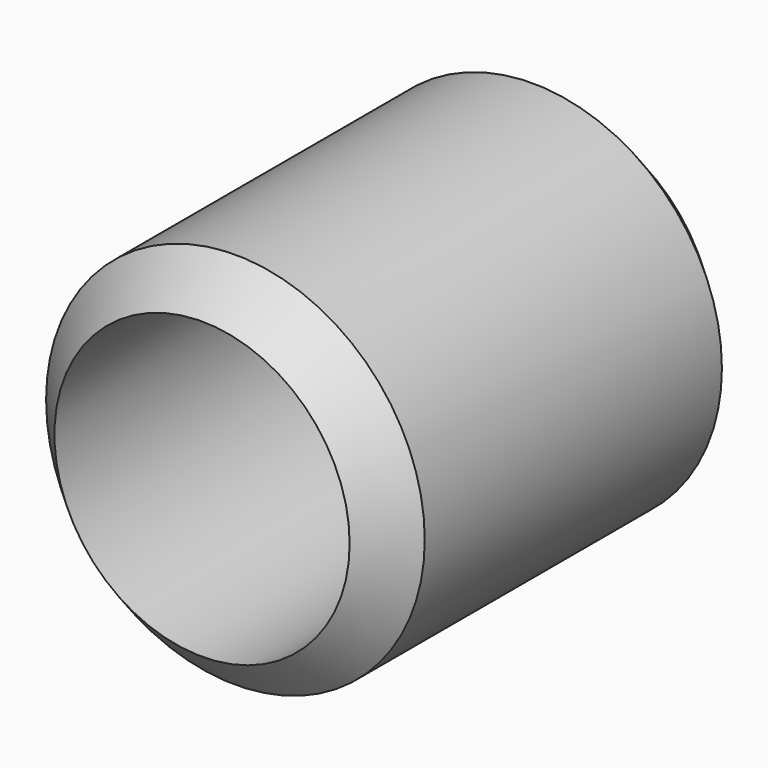
from build123d import *

# Parameters (mm, degrees)
F0_R     = 7.85
F1_DEPTH = 25.4
F3_D     = 12.24


# Not quite as in the source:
# - a fillet or chamfer that OpenCascade refuses, or shapes differently, is made with other operations: its cross-section is extruded or revolved along the edge and cut away or added


with BuildPart() as f1:
    # F0 (on Front) → F1 (new body)
    with BuildSketch(Plane.XZ):
        Circle(F0_R)
    extrude(amount=F1_DEPTH)

    # F3 (through all)
    with Locations(Plane(origin=(0, 0, 0), x_dir=(-1, 0, 0), z_dir=(0, 1, 0))):
        with Locations((0, 0)):
            Hole(F3_D / 2)

    # F4: chamfer of 5 on 1 edges, made by hand

    # F4_s1 → F4_t2 (revolve, cut)
    with BuildSketch(Plane.XY):
        Polygon((7.85, -5), (2.85, 0), (7.85, 0), align=None)
    revolve(axis=Axis((0, 0, 0), (0, -1, 0)), mode=Mode.SUBTRACT)

    # F5: chamfer of 5 on 1 edges, made by hand

    # F5_s1 → F5_t2 (revolve, cut)
    with BuildSketch(Plane.XY):
        Polygon((7.85, -20.4), (2.85, -25.4), (7.85, -25.4), align=None)
    revolve(axis=Axis((0, -25.4, 0), (0, -1, 0)), mode=Mode.SUBTRACT)


solid = f1.part
